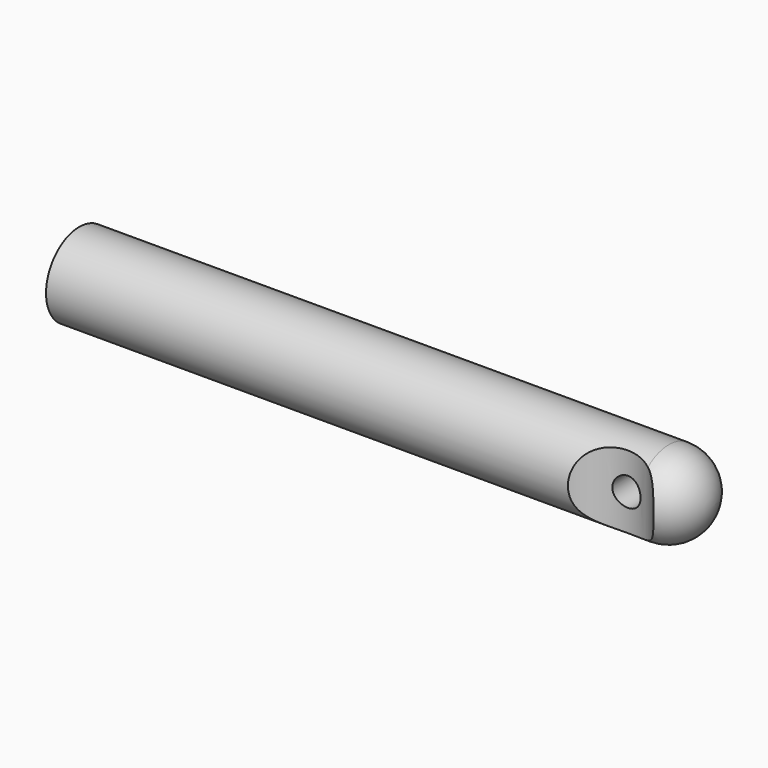
from build123d import *

# Parameters (mm, degrees)
F3_R           = 16
F4_DEPTH       = 15
F6_D           = 6.8
F6_DEPTH       = 23.75
F6_TIP         = 2.0429261047
F9_D           = 8.5
F9_START       = 2.2294414
F9_CBORE_D     = 14.25
F9_CBORE_DEPTH = 8


with BuildPart() as f2:
    # F0 (on Top) → F2 (revolve)
    with BuildSketch(Plane.XY):
        with BuildLine():
            Line((0, 12.5), (0, 0))
            Line((0, 0), (190, 0))
            ThreePointArc((190, 0), (186.3388347648, 8.8388347648), (177.5, 12.5))
            Line((177.5, 12.5), (0, 12.5))
        make_face()
    revolve(axis=Axis((6.2984433025, 0, 0), (-1, 0, 0)))

    # F3 (on Top) → F4 (cut, symmetric)
    with BuildSketch(Plane.XY):
        with Locations((170, -22)):
            Circle(F3_R)
    extrude(amount=F4_DEPTH, both=True, mode=Mode.SUBTRACT)

    # F6
    with Locations(Plane(origin=(0, 0, 0), x_dir=(0, 1, 0), z_dir=(-1, 0, 0))):
        with Locations((0, 0)):
            Hole(F6_D / 2, depth=F6_DEPTH)
            with Locations((0, 0, -(F6_DEPTH + F6_TIP / 2))):  # 118° drill point
                Cone(0, F6_D / 2, F6_TIP, mode=Mode.SUBTRACT)

    # F9 (through all)
    # its depths count from where the whole tool has entered the part; down to there all is cleared
    with Locations(Plane(origin=(0, 12.5, 0), x_dir=(1, 0, 0), z_dir=(0, 1, 0)).offset(-F9_START)):
        with Locations((170, 0)):
            CounterBoreHole(F9_D / 2, F9_CBORE_D / 2, F9_CBORE_DEPTH)


solid = f2.part
